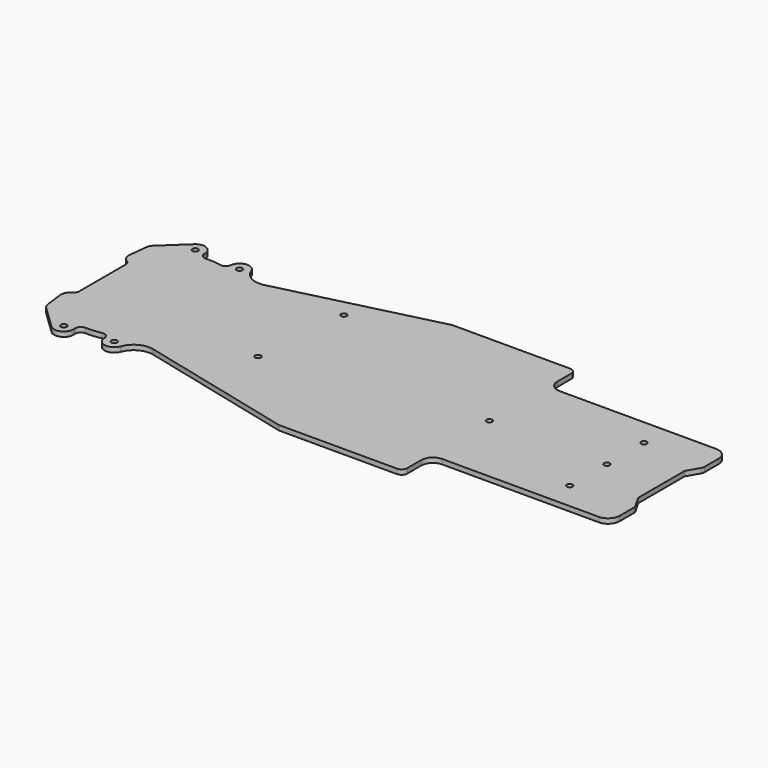
from build123d import *

# Parameters (mm, degrees)
F0_R     = 1.5
F1_DEPTH = 2.5


# Not quite as in the source:
# - ends of sketch curves that miss each other by under 0.0002 mm in the source are joined


with BuildPart() as f1:
    # F0 (on Top) → F1 (new body)
    with BuildSketch(Plane.XY):
        with BuildLine():
            ThreePointArc((148.553042, 14.928769), (146.7956826871, 19.1714096871), (142.553042, 20.928769))
            Line((142.553042, 20.928769), (61.546959, 20.928769))
            ThreePointArc((61.546959, 20.928769), (57.3043183129, 22.6861283129), (55.546959, 26.928769))
            Line((55.546959, 26.928769), (55.546959, 35.928769))
            ThreePointArc((55.546959, 35.928769), (54.6682793436, 38.0500893436), (52.546959, 38.928769))
            Line((52.546959, 38.928769), (-8.453041, 38.928769))
            Line((-8.453041, 38.928769), (-89.559124, 18.860903))
            ThreePointArc((-89.559124, 18.860903), (-96.6607350116, 19.7413862614), (-101.3556837465, 25.1419037277))
            ThreePointArc((-101.3556837465, 25.1419037277), (-106.6281165379, 28.3955877128), (-111.0175785103, 24.0232160611))
            ThreePointArc((-111.0175785103, 24.0232160611), (-112.2824719314, 21.9176106757), (-114.6963029885, 21.462694048))
            ThreePointArc((-114.6963029885, 21.462694048), (-118.4956024313, 22.0698924501), (-122.3430789933, 22.0869199077))
            ThreePointArc((-122.3430789933, 22.0869199077), (-124.651171475, 22.9272997317), (-125.557821603, 25.2101739826))
            ThreePointArc((-125.557821603, 25.2101739826), (-128.4655562478, 29.9721606196), (-133.972746844, 29.0764548336))
            Line((-133.972746844, 29.0764548336), (-145.972747, 17.826455))
            ThreePointArc((-145.972747, 17.826455), (-147.027366593, 16.4104523305), (-147.524076258, 14.7161780279))
            Line((-147.524076258, 14.7161780279), (-148.524076, 5.466178))
            ThreePointArc((-148.524076, 5.466178), (-148.0067044123, 2.6561312792), (-146.0349377658, 0.5882404096))
            ThreePointArc((-146.0349377658, 0.5882404096), (-144.929137249, -0.5106558369), (-144.524076, -2.016077))
            Line((-144.524076, -2.016077), (-144.524076, -32.126386))
            ThreePointArc((-144.524076, -32.126386), (-144.929137249, -33.6318071631), (-146.0349379189, -34.7307031419))
            ThreePointArc((-146.0349379189, -34.7307031419), (-148.0285132018, -36.8418479978), (-148.5127305604, -39.7048550716))
            Line((-148.5127305604, -39.7048550716), (-147.333918, -48.932011))
            ThreePointArc((-147.333918, -48.932011), (-146.8569609625, -50.4905877681), (-145.8877919349, -51.801068932))
            Line((-145.8877919349, -51.801068932), (-134.012517, -63.181221))
            ThreePointArc((-134.012517, -63.181221), (-128.2758744449, -64.0225805122), (-125.6012880056, -58.8783080008))
            ThreePointArc((-125.6012880056, -58.8783080008), (-124.8721529677, -56.4691107751), (-122.564742997, -55.4632638637))
            ThreePointArc((-122.564742997, -55.4632638637), (-118.5664827026, -55.3440377294), (-114.6018211423, -54.8132282387))
            ThreePointArc((-114.6018211423, -54.8132282387), (-112.1618303627, -55.4315323166), (-111.051616739, -57.6905760176))
            ThreePointArc((-111.051616739, -57.6905760176), (-106.8640436675, -62.5050200787), (-101.3556836703, -59.2843667555))
            ThreePointArc((-101.3556836703, -59.2843667555), (-96.6607350116, -53.8838492614), (-89.5591238689, -53.0033654703))
            Line((-89.5591238689, -53.0033654703), (-8.453041, -73.071231))
            Line((-8.453041, -73.071231), (52.546959, -73.071231))
            ThreePointArc((52.546959, -73.071231), (54.6682793436, -72.1925513436), (55.546959, -70.071231))
            Line((55.546959, -70.071231), (55.546959, -61.071231))
            ThreePointArc((55.546959, -61.071231), (57.3043183129, -56.8285903129), (61.546959, -55.071231))
            Line((61.546959, -55.071231), (142.553042, -55.071231))
            ThreePointArc((142.553042, -55.071231), (146.7956826871, -53.3138716871), (148.553042, -49.071231))
            Line((148.553042, -49.071231), (148.553042, -39.867925))
            ThreePointArc((148.553042, -39.867925), (148.4525408985, -39.0979210147), (148.1577712418, -38.3795078619))
            Line((148.1577712418, -38.3795078619), (144.750677, -32.417093))
            ThreePointArc((144.750677, -32.417093), (144.6032924632, -32.057886663), (144.553042, -31.672885))
            Line((144.553042, -31.672885), (144.553042, -2.469578))
            ThreePointArc((144.553042, -2.469578), (144.6032924632, -2.084576337), (144.7506770407, -1.7253700232))
            Line((144.7506770407, -1.7253700232), (148.157771, 4.237045))
            ThreePointArc((148.157771, 4.237045), (148.4525408985, 4.9554580147), (148.553042, 5.725462))
            Line((148.553042, 5.725462), (148.553042, 14.928769))
        make_face()
        with Locations((-130.553041, -59.571231)):
            Circle(F0_R, mode=Mode.SUBTRACT)
        with Locations((-106.053041, -57.571231)):
            Circle(F0_R, mode=Mode.SUBTRACT)
        with Locations((-52.553041, -31.571231)):
            Circle(F0_R, mode=Mode.SUBTRACT)
        with Locations((116.346959, -41.071231)):
            Circle(F0_R, mode=Mode.SUBTRACT)
        with Locations((-106.053041, 23.428769)):
            Circle(F0_R, mode=Mode.SUBTRACT)
        with Locations((-130.553041, 25.428769)):
            Circle(F0_R, mode=Mode.SUBTRACT)
        with Locations((-48.053041, 18.428769)):
            Circle(F0_R, mode=Mode.SUBTRACT)
        with Locations((55.546959, -17.071231)):
            Circle(F0_R, mode=Mode.SUBTRACT)
        with Locations((116.346959, -17.071231)):
            Circle(F0_R, mode=Mode.SUBTRACT)
        with Locations((116.346959, 6.928769)):
            Circle(F0_R, mode=Mode.SUBTRACT)
    extrude(amount=-F1_DEPTH)


solid = f1.part
